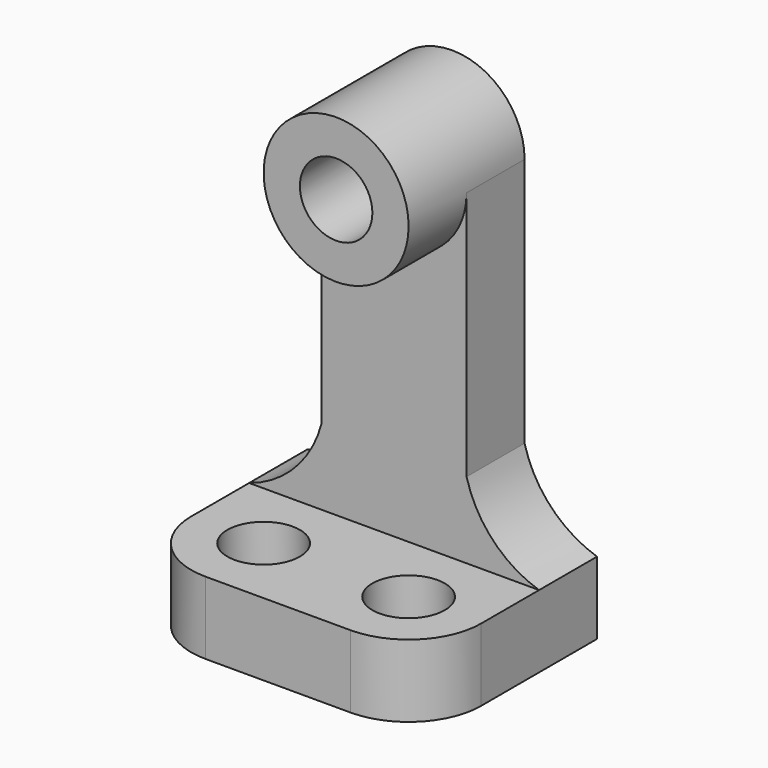
from build123d import *

# Parameters (mm, degrees)
F0_W     = 50.8
F0_H     = 38.1
F1_DEPTH = 12.7
F3_DEPTH = 12.7
F5_DEPTH = 12.7
F6_R     = 6.3499999233
F7_DEPTH = 25.401
F8_R     = 6.35
F9_DEPTH = 12.701
F10_R    = 12.7


with BuildPart() as f1:
    # F0 (on Top) → F1 (new body)
    with BuildSketch(Plane.XY):
        Rectangle(F0_W, F0_H)
    extrude(amount=F1_DEPTH)

    # F2 (on face) → F3 (join)
    with BuildSketch(Plane(origin=(0, 19.05, 0), x_dir=(-1, 0, 0), z_dir=(0, 1, 0))):
        with BuildLine():
            ThreePointArc((-12.7, 26.0490588844), (-17.3287683055, 17.7369875968), (-25.4, 12.7))
            Line((-25.4, 12.7), (-12.7, 12.7))
            Line((-12.7, 12.7), (12.7, 12.7))
            Line((12.7, 12.7), (25.4, 12.7))
            ThreePointArc((25.4, 12.7), (17.3287683055, 17.7369875968), (12.7, 26.0490588844))
            Line((12.7, 26.0490588844), (12.7, 69.85))
            ThreePointArc((12.7, 69.85), (0, 57.15), (-12.7, 69.85))
            Line((-12.7, 69.85), (-12.7, 26.0490588844))
        make_face()
        with BuildLine():
            ThreePointArc((12.7, 69.85), (0, 82.55), (-12.7, 69.85))
            ThreePointArc((-12.7, 69.85), (0, 57.15), (12.7, 69.85))
        make_face()
    extrude(amount=-F3_DEPTH)

    # F4 (on face) → F5 (join)
    with BuildSketch(Plane.XZ.offset(-6.35)):
        with BuildLine():
            ThreePointArc((-12.7, 69.85), (0, 57.15), (12.7, 69.85))
            ThreePointArc((12.7, 69.85), (0, 82.55), (-12.7, 69.85))
        make_face()
    extrude(amount=F5_DEPTH)

    # F6 (on face) → F7 (cut, through all)
    with BuildSketch(Plane.XZ.offset(6.35)):
        with Locations((0, 69.85)):
            Circle(F6_R)
    extrude(amount=-F7_DEPTH, mode=Mode.SUBTRACT)

    # F8 (on face) → F9 (cut, through all)
    with BuildSketch(Plane.XY.offset(12.7)):
        with Locations((-12.7, -6.35)):
            Circle(F8_R)
        with Locations((12.7, -6.35)):
            Circle(F8_R)
    extrude(amount=-F9_DEPTH, mode=Mode.SUBTRACT)

    # F10
    f10_edges = [f1.edges().sort_by_distance(p)[0] for p in [
        (-25.4, -19.05, 6.35),
        (25.4, -19.05, 6.35),
    ]]
    fillet(f10_edges, radius=F10_R)


solid = f1.part
